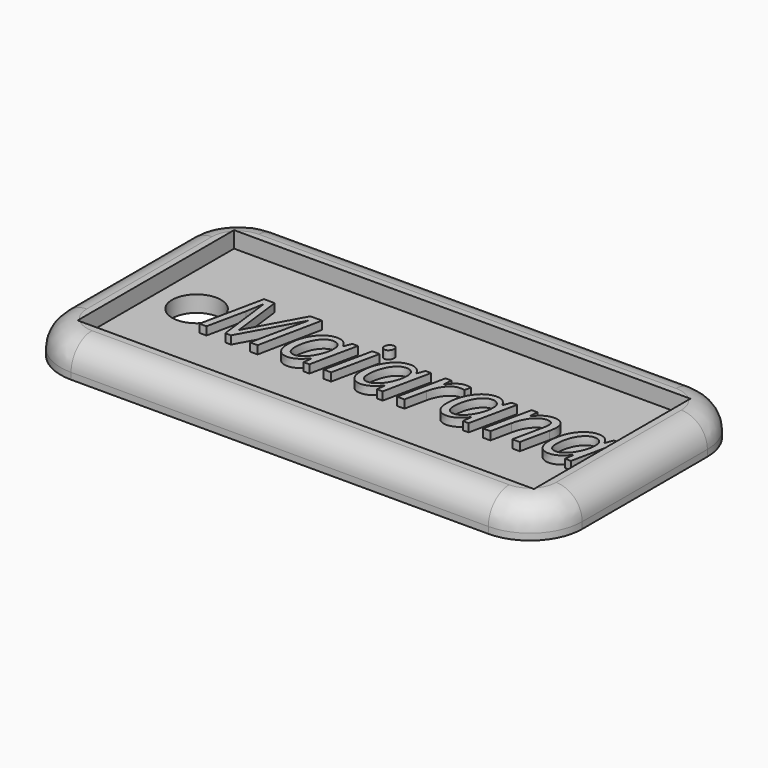
from build123d import *

# Parameters (mm, degrees)
F0_W         = 44.45
F0_H         = 19.05
F0_R         = 2.38125
F1_DEPTH     = 1.5875
F0_W_2       = 50.8
F0_H_2       = 25.4
F2_DEPTH     = 3.175
F3_R         = 5.08
F4_T1_DEPTH  = 40.64
F4_T3_DEPTH  = 15.24
F4_T6_ANGLE  = 90
F4_T8_ANGLE  = 90
F4_T10_ANGLE = 90
F4_T12_ANGLE = 90
F5_TEXT_SIZE = 8.7172887173
F6_DEPTH     = 0.79375


# Not quite as in the source:
# - a fillet or chamfer that OpenCascade refuses, or shapes differently, is made with other operations: its cross-section is extruded or revolved along the edge and cut away or added
# - a length typed as a fraction of an inch, garbled in the dataset ("3 / 203.2 mm" for 3/8 in), is restored
# - Text() gives the source's letters only with a copy of the font that has no kerning and outlines rounded to 1/6400 em; it was checked with that copy


with BuildPart() as f1:
    # F0 (on Top) → F1 (new body)
    with BuildSketch(Plane.XY):
        with Locations((25.4, 12.7)):
            Rectangle(F0_W, F0_H)
        with Locations((7.14375, 12.7)):
            Circle(F0_R, mode=Mode.SUBTRACT)
    extrude(amount=F1_DEPTH)

    # F0 (on Top) → F2 (join)
    with BuildSketch(Plane.XY):
        with Locations((25.4, 12.7)):
            Rectangle(F0_W_2, F0_H_2)
        with Locations((25.4, 12.7)):
            Rectangle(F0_W, F0_H, mode=Mode.SUBTRACT)
    extrude(amount=F2_DEPTH)

    # F3
    f3_edges = [f1.edges().sort_by_distance(p)[0] for p in [
        (50.8, 0, 1.5875),
        (0, 0, 1.5875),
        (50.8, 25.4, 1.5875),
        (0, 25.4, 1.5875),
    ]]
    fillet(f3_edges, radius=F3_R)

    # F4: fillet of radius 2.54 on 8 edges, made by hand

    # F4_s2 → F4_t1 (cut)
    with BuildSketch(Plane.YZ.offset(5.08)):
        with BuildLine():
            ThreePointArc((25.4, 0.635), (24.6560512242, 2.4310512242), (22.86, 3.175))
            Line((22.86, 3.175), (25.4, 3.175))
            Line((25.4, 3.175), (25.4, 0.635))
        make_face()
        with BuildLine():
            ThreePointArc((0, 0.635), (0.7439487758, 2.4310512242), (2.54, 3.175))
            Line((2.54, 3.175), (0, 3.175))
            Line((0, 3.175), (0, 0.635))
        make_face()
    extrude(amount=F4_T1_DEPTH, mode=Mode.SUBTRACT)

    # F4_s4 → F4_t3 (cut)
    with BuildSketch(Plane.XZ.offset(-20.32)):
        with BuildLine():
            ThreePointArc((0, 0.635), (0.7439487758, 2.4310512242), (2.54, 3.175))
            Line((2.54, 3.175), (0, 3.175))
            Line((0, 3.175), (0, 0.635))
        make_face()
        with BuildLine():
            ThreePointArc((50.8, 0.635), (50.0560512242, 2.4310512242), (48.26, 3.175))
            Line((48.26, 3.175), (50.8, 3.175))
            Line((50.8, 3.175), (50.8, 0.635))
        make_face()
    extrude(amount=F4_T3_DEPTH, mode=Mode.SUBTRACT)

    # F4_s5 → F4_t6 (revolve, cut)
    with BuildSketch(Plane.XZ.offset(-20.32)):
        with BuildLine():
            ThreePointArc((0, 0.635), (0.7439487758, 2.4310512242), (2.54, 3.175))
            Line((2.54, 3.175), (0, 3.175))
            Line((0, 3.175), (0, 0.635))
        make_face()
    revolve(axis=Axis((5.08, 20.32, 3.175), (0, 0, -1)), revolution_arc=F4_T6_ANGLE, mode=Mode.SUBTRACT)

    # F4_s7 → F4_t8 (revolve, cut)
    with BuildSketch(Plane.XZ.offset(-5.08)):
        with BuildLine():
            ThreePointArc((0, 0.635), (0.7439487758, 2.4310512242), (2.54, 3.175))
            Line((2.54, 3.175), (0, 3.175))
            Line((0, 3.175), (0, 0.635))
        make_face()
    revolve(axis=Axis((5.08, 5.08, 3.175), (0, 0, 1)), revolution_arc=F4_T8_ANGLE, mode=Mode.SUBTRACT)

    # F4_s9 → F4_t10 (revolve, cut)
    with BuildSketch(Plane.XZ.offset(-20.32)):
        with BuildLine():
            ThreePointArc((50.8, 0.635), (50.0560512242, 2.4310512242), (48.26, 3.175))
            Line((48.26, 3.175), (50.8, 3.175))
            Line((50.8, 3.175), (50.8, 0.635))
        make_face()
    revolve(axis=Axis((45.72, 20.32, 3.175), (0, 0, 1)), revolution_arc=F4_T10_ANGLE, mode=Mode.SUBTRACT)

    # F4_s11 → F4_t12 (revolve, cut)
    with BuildSketch(Plane.YZ.offset(45.72)):
        with BuildLine():
            ThreePointArc((0, 0.635), (0.7439487758, 2.4310512242), (2.54, 3.175))
            Line((2.54, 3.175), (0, 3.175))
            Line((0, 3.175), (0, 0.635))
        make_face()
    revolve(axis=Axis((45.72, 5.08, 3.175), (0, 0, 1)), revolution_arc=F4_T12_ANGLE, mode=Mode.SUBTRACT)

    # F5 (on face) → F6 (join)
    with BuildSketch(Plane.XY.offset(1.5875)):
        with Locations((9.432845674, 9.7341442645)):
            Text('Maiarana', F5_TEXT_SIZE, font='Open Sans', font_style=FontStyle.ITALIC, text_align=(TextAlign.LEFT, TextAlign.BOTTOM))
    extrude(amount=F6_DEPTH)


solid = f1.part
